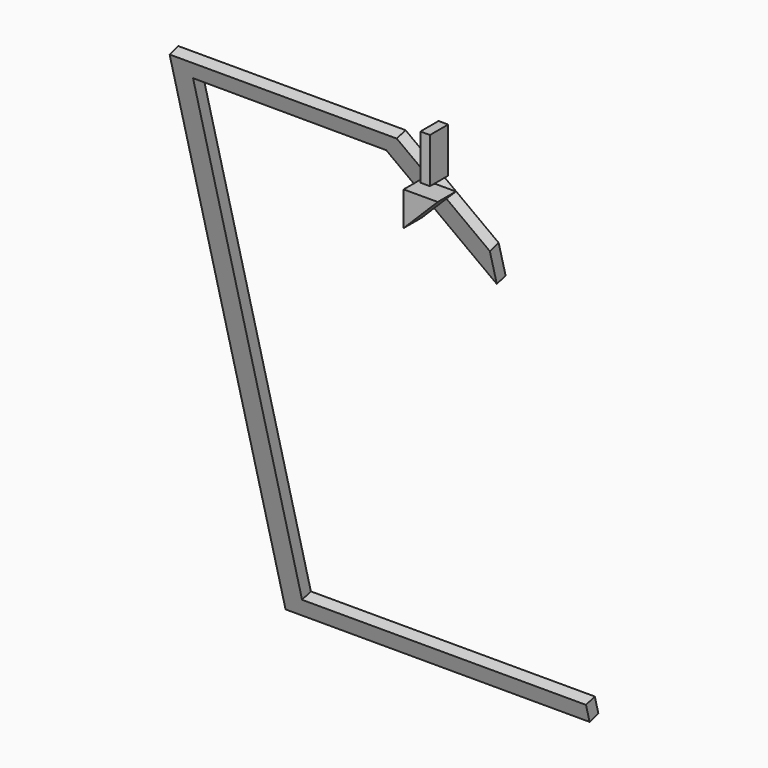
from build123d import *

# Parameters (mm, degrees)
F1_DEPTH     = 1.27
F2_ANGLE     = 15
F3_TEXT_SIZE = 14.1111111111
F4_DEPTH     = 5.08


# Not quite as in the source:
# - Text() gives the source's letters only with a copy of the font that has no kerning and outlines rounded to 1/6400 em; it was checked with that copy


with BuildPart() as f1:
    # F0 (on Front) → F1 (new body, symmetric)
    with BuildSketch(Plane.XZ):
        Polygon((12.9832137386, 50.2433507582), (-3.818668965, 69.6376003378), (-54.618668965, 69.6376003378), (-55.0108218024, -57.3617942125), (12.9832137386, -57.3617942125), (12.9832137386, -53.4648511343), (-50.5167862614, -53.4648511343), (-50.1481625942, 65.914579743), (-6.9683684471, 65.7812477783), (12.9832137386, 42.7385750104), align=None)
    extrude(amount=F1_DEPTH, both=True)


with BuildPart() as f1_1:
    # F2: moved
    add(f1.part.rotate(Axis((-28.5582655206, 0, 65.8479137606), (0.9999952327, 0, -0.0030878176)), F2_ANGLE))

    # F3 (on Front) → F4 (join)
    with BuildSketch(Plane.XZ):
        Polygon((7.62, 61.5777534187), (0, 61.5777534187), (0, 53.9577534187), align=None)
        with Locations((2.4788761511, 64.117744565)):
            Text('I', F3_TEXT_SIZE, font='Open Sans', font_style=FontStyle.BOLD, text_align=(TextAlign.LEFT, TextAlign.BOTTOM))
    extrude(amount=F4_DEPTH)


solid = f1_1.part
